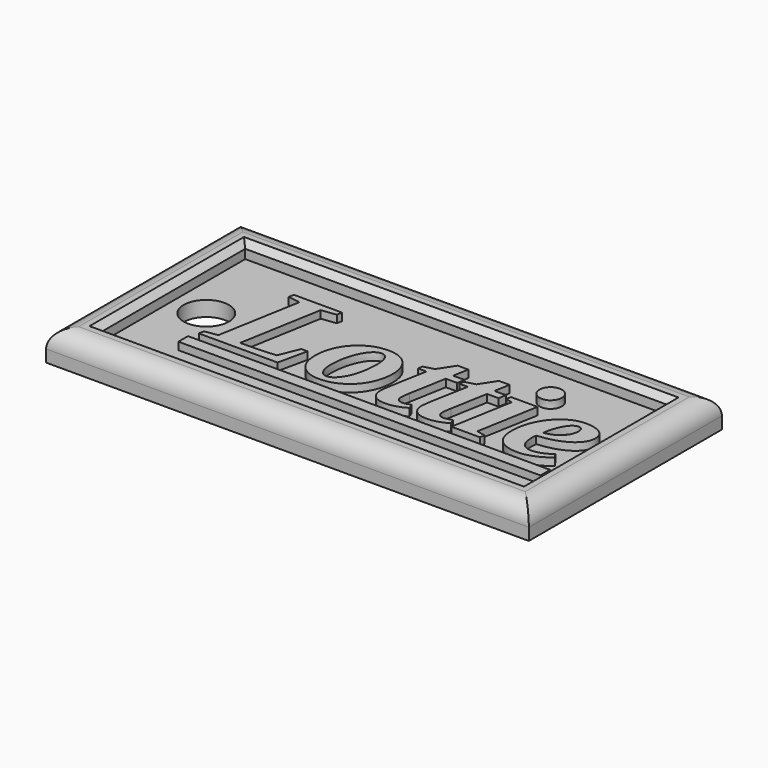
from build123d import *

# Parameters (mm, degrees)
F0_W         = 44.45
F0_H         = 19.05
F0_R         = 2.38125
F1_DEPTH     = 1.5875
F0_W_2       = 50.8
F0_H_2       = 25.4
F2_DEPTH     = 3.175
F3_W         = 38.1
F3_H         = 1.2653651647
F3_TEXT_SIZE = 15.6407953817
F4_DEPTH     = 0.79375
F5_R         = 1.905
F6_SIZE      = 0.635


# Not quite as in the source:
# - Text() gives the source's letters only with a copy of the font that has no kerning and outlines rounded to 1/6400 em; it was checked with that copy


with BuildPart() as f1:
    # F0 (on Top) → F1 (new body)
    with BuildSketch(Plane.XY):
        with Locations((25.4, 12.7)):
            Rectangle(F0_W, F0_H)
        with Locations((6.69925, 12.7)):
            Circle(F0_R, mode=Mode.SUBTRACT)
    extrude(amount=F1_DEPTH)

    # F0 (on Top) → F2 (join)
    with BuildSketch(Plane.XY):
        with Locations((25.4, 12.7)):
            Rectangle(F0_W_2, F0_H_2)
        with Locations((25.4, 12.7)):
            Rectangle(F0_W, F0_H, mode=Mode.SUBTRACT)
    extrude(amount=F2_DEPTH)

    # F3 (on face) → F4 (join)
    with BuildSketch(Plane.XY.offset(1.5875)):
        with Locations((28.067, 6.7648354452)):
            Rectangle(F3_W, F3_H)
        with Locations((9.525, 8.3294717992)):
            Text('Lottie', F3_TEXT_SIZE, font='Tinos', font_style=FontStyle.BOLDITALIC, text_align=(TextAlign.LEFT, TextAlign.BOTTOM))
    extrude(amount=F4_DEPTH)

    # F5
    f5_edges = [f1.edges().sort_by_distance(p)[0] for p in [
        (25.4, 0, 3.175),
        (0, 12.7, 3.175),
        (25.4, 25.4, 3.175),
        (50.8, 12.7, 3.175),
    ]]
    fillet(f5_edges, radius=F5_R)

    # F6
    f6_edges = [f1.edges().sort_by_distance(p)[0] for p in [
        (25.4, 22.225, 3.175),
        (47.625, 12.7, 3.175),
        (25.4, 3.175, 3.175),
        (3.175, 12.7, 3.175),
    ]]
    chamfer(f6_edges, length=F6_SIZE)


solid = f1.part
